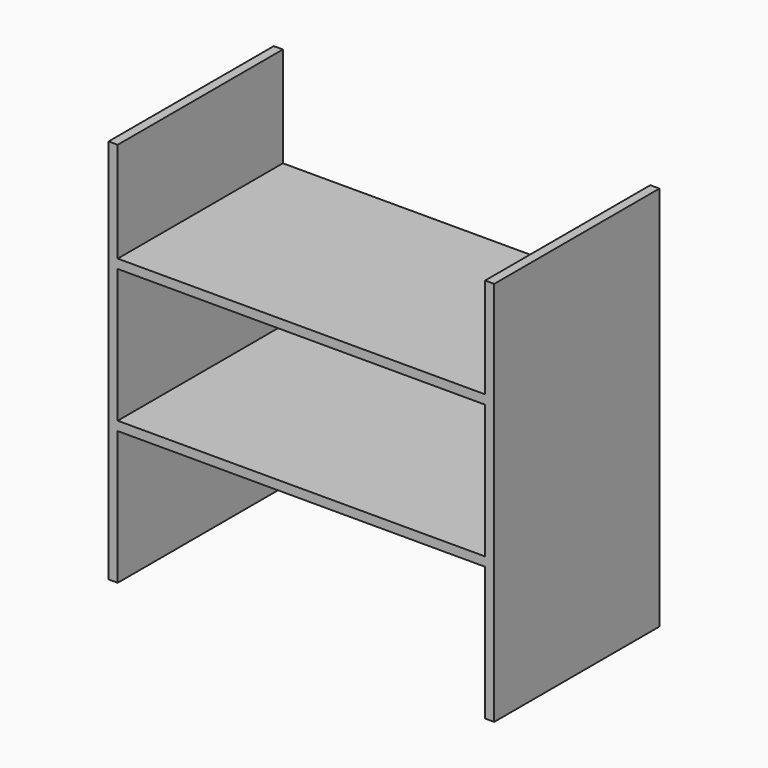
from build123d import *

# Parameters (mm, degrees)
F0_W     = 19.05
F0_H     = 19.05
F0_H_2   = 190.5
F0_H_3   = 279.4
F1_DEPTH = 431.8


with BuildPart() as f1:
    # F0 (on Front) → F1 (new body)
    with BuildSketch(Plane.XZ):
        with Locations((-393.7, 400.9142230511)):
            Rectangle(F0_W, F0_H)
        with Locations((-393.7, 296.1392230511)):
            Rectangle(F0_W, F0_H_2)
        with Locations((393.7, 400.9142230511)):
            Rectangle(F0_W, F0_H)
        with Locations((-393.7, 191.3642230511)):
            Rectangle(F0_W, F0_H)
        with Locations((393.7, 296.1392230511)):
            Rectangle(F0_W, F0_H_2)
        Polygon((-162.0973050594, 200.8892230511), (-384.175, 200.8892230511), (-384.175, 181.8392230511), (-162.0973050594, 181.8392230511), (384.175, 181.8392230511), (384.175, 200.8892230511), align=None)
        with Locations((-393.7, 42.1392230511)):
            Rectangle(F0_W, F0_H_3)
        with Locations((393.7, 191.3642230511)):
            Rectangle(F0_W, F0_H)
        with Locations((-393.7, -107.0857769489)):
            Rectangle(F0_W, F0_H)
        with Locations((393.7, 42.1392230511)):
            Rectangle(F0_W, F0_H_3)
        Polygon((-162.0973050594, -97.5607769489), (-384.175, -97.5607769489), (-384.175, -116.6107769489), (-162.0973050594, -116.6107769489), (384.175, -116.6107769489), (384.175, -97.5607769489), align=None)
        with Locations((-393.7, -256.3107769489)):
            Rectangle(F0_W, F0_H_3)
        with Locations((393.7, -107.0857769489)):
            Rectangle(F0_W, F0_H)
        with Locations((393.7, -256.3107769489)):
            Rectangle(F0_W, F0_H_3)
    extrude(amount=-F1_DEPTH)


solid = f1.part
